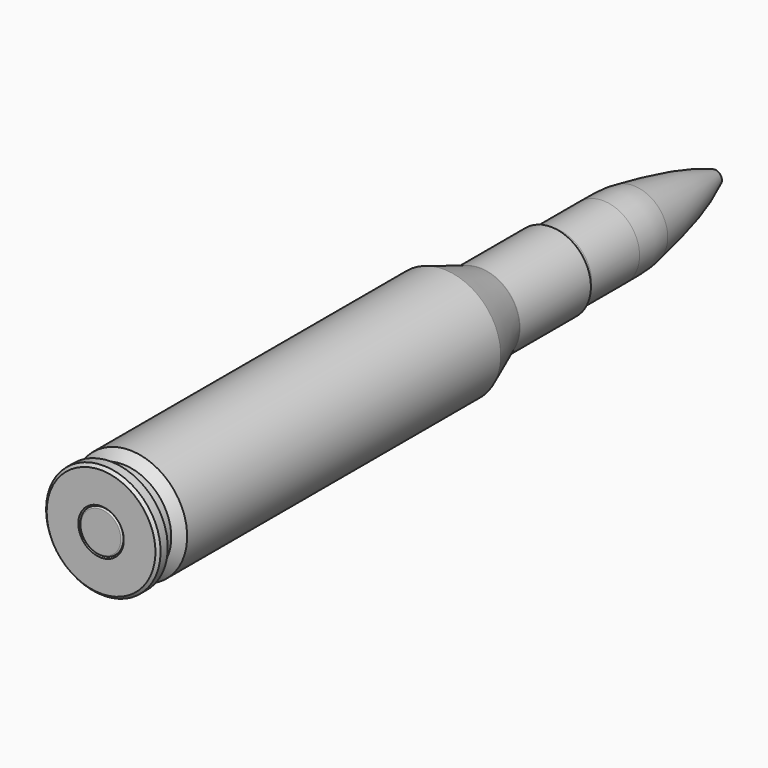
from build123d import *

# Parameters (mm, degrees)
F3_DEPTH = 5.3848
F4_R     = 0.254
F5_SIZE  = 0.508


# Not quite as in the source:
# - a fillet or chamfer that OpenCascade refuses, or shapes differently, is made with other operations: its cross-section is extruded or revolved along the edge and cut away or added


with BuildPart() as f1:
    # F0 (on Top) → F1 (revolve)
    with BuildSketch(Plane.XY):
        Polygon((-19.1289222062, -69.1020740439), (-15.3252963252, -69.1020740439), (-15.3252963252, 26.1417003232), (-21.4466963252, 26.1417003232), (-22.4372963252, 26.1417003232), (-22.4372963252, 10.0381003232), (-25.5360963252, 1.9012442353), (-25.5360963252, -68.0084118526), (-23.9612963252, -69.5832118526), (-23.9612963252, -72.3429557647), (-25.5360963252, -72.3429557647), (-25.5360963252, -74.4511557647), (-19.1289222062, -74.4511557647), align=None)
        with BuildLine():
            Line((-21.4466963252, 26.1417003232), (-15.3252963252, 26.1417003232))
            Line((-15.3252963252, 26.1417003232), (-15.3252963252, 62.7088442353))
            Line((-15.3252963252, 62.7088442353), (-15.3863094747, 62.7088442353))
            add(Edge.make_bspline(
                [(-15.3863094747, 62.7088442353), (-16.22922346, 62.7838820219), (-16.4167433977, 62.5745207071), (-16.5730696172, 62.435567379)],
                knots=[0, 0, 0, 0, 1.2178176694, 1.2178176694, 1.2178176694, 1.2178176694], degree=3))
            add(Edge.make_bspline(
                [(-16.5730696172, 62.435567379), (-19.0194975585, 56.8844638765), (-20.2809497714, 50.9883202612), (-21.4389152825, 44.2740693688)],
                knots=[0, 0, 0, 0, 18.8020335074, 18.8020335074, 18.8020335074, 18.8020335074], degree=3))
            add(Edge.make_bspline(
                [(-21.8475367874, 37.4826304615), (-21.8703859069, 39.438161999), (-21.8947399408, 42.3613935709), (-21.4389152825, 44.2740693688)],
                knots=[0, 0, 0, 0, 6.8037205974, 6.8037205974, 6.8037205974, 6.8037205974], degree=3))
            Line((-21.8475367874, 37.4826304615), (-21.8475367874, 26.8227737397))
            add(Edge.make_bspline(
                [(-21.8475367874, 26.8227737397), (-21.8473226346, 26.2848939747), (-21.9419963252, 26.1417003232), (-21.4466963252, 26.1417003232)],
                knots=[0, 0, 0, 0, 0.7902746831, 0.7902746831, 0.7902746831, 0.7902746831], degree=3))
        make_face()
    revolve(axis=Axis((-15.3252963252, -24.1547277207, 0), (0, 1, 0)))

    # F2: chamfer of 0.254 on 3 edges, made by hand

    # F2_s1 → F2_t2 (revolve)
    with BuildSketch(Plane.XY):
        Polygon((-22.4372963252, 10.0848293801), (-22.4539271766, 9.9944308884), (-22.4372963252, 10.0381003232), align=None)
    revolve(axis=Axis((-15.3252963252, 10.0381003232, 0), (0, 1, 0)))

    # F2_s3 → F2_t4 (revolve, cut)
    with BuildSketch(Plane.XY):
        Polygon((-19.1289222062, -74.1971557647), (-19.3829222062, -74.4511557647), (-19.1289222062, -74.4511557647), align=None)
    revolve(axis=Axis((-15.3252963252, -74.4511557647, 0), (0, 1, 0)), mode=Mode.SUBTRACT)

    # F2_s5 → F2_t6 (revolve, cut)
    with BuildSketch(Plane.XY):
        Polygon((-22.4372963252, 25.8877003232), (-22.1832963252, 26.1417003232), (-22.4372963252, 26.1417003232), align=None)
    revolve(axis=Axis((-15.3252963252, 26.1417003232, 0), (0, 1, 0)), mode=Mode.SUBTRACT)

    # F3 (add): a face of the model
    f3_faces = [f1.faces().sort_by_distance(p)[0] for p in [
        (-15.3252963252, -69.1020740439, 0),
    ]]
    extrude(f3_faces, amount=F3_DEPTH)

    # F4
    f4_edges = [f1.edges().sort_by_distance(p)[0] for p in [
        (-11.52167, -74.486874, 0),
    ]]
    fillet(f4_edges, radius=F4_R)

    # F5
    f5_edges = [f1.edges().sort_by_distance(p)[0] for p in [
        (-5.114496, -74.451156, 0),
    ]]
    chamfer(f5_edges, length=F5_SIZE)


solid = f1.part
